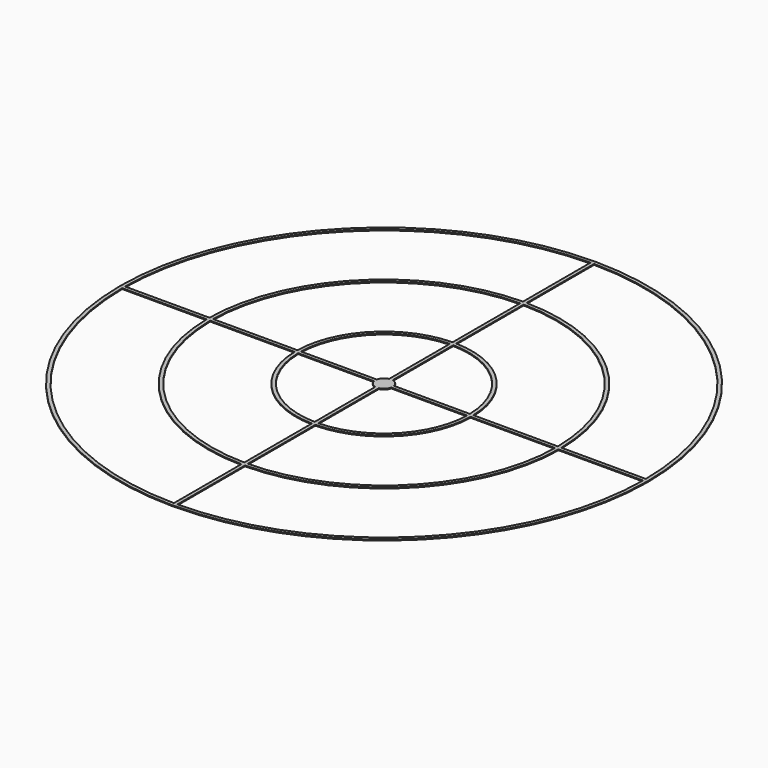
from build123d import *

# Parameters (mm, degrees)
F1_DEPTH = 0.25


with BuildPart() as f1:
    # F0 (on Top) → F1 (new body)
    with BuildSketch(Plane.XY):
        with BuildLine():
            ThreePointArc((-0.5, -73.9983107915), (-52.3259018078, -52.3259018078), (-73.9983107915, -0.5))
            Line((-73.9983107915, -0.5), (-49.9974999375, -0.5))
            Line((-49.9974999375, -0.5), (-48.9974489132, -0.5))
            ThreePointArc((-48.9974489132, -0.5), (-49, 0), (-48.9974489132, 0.5))
            ThreePointArc((-48.9974489132, 0.5), (-34.6482322781, 34.6482322781), (-0.5, 48.9974489132))
            Line((-0.5, 48.9974489132), (-0.5, 49.9974999375))
            ThreePointArc((-0.5, 49.9974999375), (-35.3553390593, 35.3553390593), (-49.9974999375, 0.5))
            Line((-49.9974999375, 0.5), (-73.9983107915, 0.5))
            ThreePointArc((-73.9983107915, 0.5), (-52.3259018078, 52.3259018078), (-0.5, 73.9983107915))
            Line((-0.5, 73.9983107915), (-0.5, 74.9983333148))
            ThreePointArc((-0.5, 74.9983333148), (-53.033008589, 53.033008589), (-74.9983333148, 0.5))
            Line((-74.9983333148, 0.5), (-74.9983333148, -0.5))
            ThreePointArc((-74.9983333148, -0.5), (-53.033008589, -53.033008589), (-0.5, -74.9983333148))
            Line((-0.5, -74.9983333148), (-0.5, -73.9983107915))
        make_face()
        with BuildLine():
            Line((-0.5, -49.9974999375), (-0.5, -73.9983107915))
            ThreePointArc((-0.5, -73.9983107915), (0, -74), (0.5, -73.9983107915))
            Line((0.5, -73.9983107915), (0.5, -49.9974999375))
            ThreePointArc((0.5, -49.9974999375), (0, -50), (-0.5, -49.9974999375))
        make_face()
        with BuildLine():
            ThreePointArc((0.5, -73.9983107915), (0, -74), (-0.5, -73.9983107915))
            Line((-0.5, -73.9983107915), (-0.5, -74.9983333148))
            Line((-0.5, -74.9983333148), (0.5, -74.9983333148))
            Line((0.5, -74.9983333148), (0.5, -73.9983107915))
        make_face()
        with BuildLine():
            Line((-48.9974489132, -0.5), (-49.9974999375, -0.5))
            ThreePointArc((-49.9974999375, -0.5), (-35.3553390593, -35.3553390593), (-0.5, -49.9974999375))
            ThreePointArc((-0.5, -49.9974999375), (0, -50), (0.5, -49.9974999375))
            Line((0.5, -49.9974999375), (0.5, -48.9974489132))
            ThreePointArc((0.5, -48.9974489132), (0, -49), (-0.5, -48.9974489132))
            ThreePointArc((-0.5, -48.9974489132), (-34.6482322781, -34.6482322781), (-48.9974489132, -0.5))
        make_face()
        with BuildLine():
            ThreePointArc((73.9983107915, -0.5), (52.3259018078, -52.3259018078), (0.5, -73.9983107915))
            Line((0.5, -73.9983107915), (0.5, -74.9983333148))
            ThreePointArc((0.5, -74.9983333148), (53.033008589, -53.033008589), (74.9983333148, -0.5))
            Line((74.9983333148, -0.5), (73.9983107915, -0.5))
        make_face()
        with BuildLine():
            ThreePointArc((-48.9974489132, 0.5), (-49, 0), (-48.9974489132, -0.5))
            Line((-48.9974489132, -0.5), (-24.9949994999, -0.5))
            Line((-24.9949994999, -0.5), (-23.9947911014, -0.5))
            ThreePointArc((-23.9947911014, -0.5), (-24, 0), (-23.9947911014, 0.5))
            ThreePointArc((-23.9947911014, 0.5), (-16.9705627485, 16.9705627485), (-0.5, 23.9947911014))
            Line((-0.5, 23.9947911014), (-0.5, 24.9949994999))
            ThreePointArc((-0.5, 24.9949994999), (-17.6776695297, 17.6776695297), (-24.9949994999, 0.5))
            Line((-24.9949994999, 0.5), (-48.9974489132, 0.5))
        make_face()
        with BuildLine():
            Line((49.9974999375, -0.5), (73.9983107915, -0.5))
            ThreePointArc((73.9983107915, -0.5), (74, 0), (73.9983107915, 0.5))
            Line((73.9983107915, 0.5), (49.9974999375, 0.5))
            ThreePointArc((49.9974999375, 0.5), (50, 0), (49.9974999375, -0.5))
        make_face()
        with BuildLine():
            ThreePointArc((73.9983107915, 0.5), (74, 0), (73.9983107915, -0.5))
            Line((73.9983107915, -0.5), (74.9983333148, -0.5))
            Line((74.9983333148, -0.5), (74.9983333148, 0.5))
            Line((74.9983333148, 0.5), (73.9983107915, 0.5))
        make_face()
        with BuildLine():
            Line((0.5, -48.9974489132), (0.5, -49.9974999375))
            ThreePointArc((0.5, -49.9974999375), (35.3553390593, -35.3553390593), (49.9974999375, -0.5))
            Line((49.9974999375, -0.5), (48.9974489132, -0.5))
            ThreePointArc((48.9974489132, -0.5), (34.6482322781, -34.6482322781), (0.5, -48.9974489132))
        make_face()
        with BuildLine():
            ThreePointArc((-74.9983333148, 0.5), (-75, 0), (-74.9983333148, -0.5))
            Line((-74.9983333148, -0.5), (-74.9983333148, 0.5))
        make_face()
        with BuildLine():
            Line((-23.9947911014, -0.5), (-24.9949994999, -0.5))
            ThreePointArc((-24.9949994999, -0.5), (-17.6776695297, -17.6776695297), (-0.5, -24.9949994999))
            Line((-0.5, -24.9949994999), (-0.5, -48.9974489132))
            ThreePointArc((-0.5, -48.9974489132), (0, -49), (0.5, -48.9974489132))
            Line((0.5, -48.9974489132), (0.5, -24.9949994999))
            Line((0.5, -24.9949994999), (0.5, -23.9947911014))
            Line((0.5, -23.9947911014), (0.5, -2.4494897428))
            Line((0.5, -2.4494897428), (0.5, -0.5))
            Line((0.5, -0.5), (2.4494897428, -0.5))
            Line((2.4494897428, -0.5), (23.9947911014, -0.5))
            Line((23.9947911014, -0.5), (24.9949994999, -0.5))
            ThreePointArc((24.9949994999, -0.5), (25, 0), (24.9949994999, 0.5))
            Line((24.9949994999, 0.5), (23.9947911014, 0.5))
            Line((23.9947911014, 0.5), (2.4494897428, 0.5))
            Line((2.4494897428, 0.5), (0.5, 0.5))
            Line((0.5, 0.5), (-0.5, 0.5))
            Line((-0.5, 0.5), (-0.5, -0.5))
            Line((-0.5, -0.5), (-0.5, -2.4494897428))
            Line((-0.5, -2.4494897428), (-0.5, -23.9947911014))
            ThreePointArc((-0.5, -23.9947911014), (-16.9705627485, -16.9705627485), (-23.9947911014, -0.5))
        make_face()
        with BuildLine():
            ThreePointArc((0.5, 73.9983107915), (52.3259018078, 52.3259018078), (73.9983107915, 0.5))
            Line((73.9983107915, 0.5), (74.9983333148, 0.5))
            ThreePointArc((74.9983333148, 0.5), (53.033008589, 53.033008589), (0.5, 74.9983333148))
            Line((0.5, 74.9983333148), (0.5, 73.9983107915))
        make_face()
        with BuildLine():
            Line((48.9974489132, -0.5), (49.9974999375, -0.5))
            ThreePointArc((49.9974999375, -0.5), (50, 0), (49.9974999375, 0.5))
            Line((49.9974999375, 0.5), (48.9974489132, 0.5))
            ThreePointArc((48.9974489132, 0.5), (49, 0), (48.9974489132, -0.5))
        make_face()
        with BuildLine():
            Line((-0.5, 49.9974999375), (-0.5, 48.9974489132))
            ThreePointArc((-0.5, 48.9974489132), (0, 49), (0.5, 48.9974489132))
            Line((0.5, 48.9974489132), (0.5, 49.9974999375))
            ThreePointArc((0.5, 49.9974999375), (0, 50), (-0.5, 49.9974999375))
        make_face()
        with BuildLine():
            ThreePointArc((0.5, 48.9974489132), (0, 49), (-0.5, 48.9974489132))
            Line((-0.5, 48.9974489132), (-0.5, 24.9949994999))
            Line((-0.5, 24.9949994999), (-0.5, 23.9947911014))
            ThreePointArc((-0.5, 23.9947911014), (0, 24), (0.5, 23.9947911014))
            ThreePointArc((0.5, 23.9947911014), (16.9705627485, 16.9705627485), (23.9947911014, 0.5))
            Line((23.9947911014, 0.5), (24.9949994999, 0.5))
            ThreePointArc((24.9949994999, 0.5), (17.6776695297, 17.6776695297), (0.5, 24.9949994999))
            Line((0.5, 24.9949994999), (0.5, 48.9974489132))
        make_face()
        with BuildLine():
            ThreePointArc((-23.9947911014, 0.5), (-24, 0), (-23.9947911014, -0.5))
            Line((-23.9947911014, -0.5), (-2.4494897428, -0.5))
            Line((-2.4494897428, -0.5), (-0.5, -0.5))
            Line((-0.5, -0.5), (-0.5, 0.5))
            Line((-0.5, 0.5), (-2.4494897428, 0.5))
            Line((-2.4494897428, 0.5), (-23.9947911014, 0.5))
        make_face()
        with BuildLine():
            Line((0.5, 49.9974999375), (0.5, 73.9983107915))
            ThreePointArc((0.5, 73.9983107915), (0, 74), (-0.5, 73.9983107915))
            Line((-0.5, 73.9983107915), (-0.5, 49.9974999375))
            ThreePointArc((-0.5, 49.9974999375), (0, 50), (0.5, 49.9974999375))
        make_face()
        with BuildLine():
            ThreePointArc((-0.5, 73.9983107915), (0, 74), (0.5, 73.9983107915))
            Line((0.5, 73.9983107915), (0.5, 74.9983333148))
            Line((0.5, 74.9983333148), (-0.5, 74.9983333148))
            Line((-0.5, 74.9983333148), (-0.5, 73.9983107915))
        make_face()
        with BuildLine():
            Line((48.9974489132, 0.5), (49.9974999375, 0.5))
            ThreePointArc((49.9974999375, 0.5), (35.3553390593, 35.3553390593), (0.5, 49.9974999375))
            Line((0.5, 49.9974999375), (0.5, 48.9974489132))
            ThreePointArc((0.5, 48.9974489132), (34.6482322781, 34.6482322781), (48.9974489132, 0.5))
        make_face()
        with BuildLine():
            Line((24.9949994999, -0.5), (48.9974489132, -0.5))
            ThreePointArc((48.9974489132, -0.5), (49, 0), (48.9974489132, 0.5))
            Line((48.9974489132, 0.5), (24.9949994999, 0.5))
            ThreePointArc((24.9949994999, 0.5), (25, 0), (24.9949994999, -0.5))
        make_face()
        with BuildLine():
            Line((0.5, -23.9947911014), (0.5, -24.9949994999))
            ThreePointArc((0.5, -24.9949994999), (17.6776695297, -17.6776695297), (24.9949994999, -0.5))
            Line((24.9949994999, -0.5), (23.9947911014, -0.5))
            ThreePointArc((23.9947911014, -0.5), (16.9705627485, -16.9705627485), (0.5, -23.9947911014))
        make_face()
        with BuildLine():
            ThreePointArc((0.5, 74.9983333148), (0, 75), (-0.5, 74.9983333148))
            Line((-0.5, 74.9983333148), (0.5, 74.9983333148))
        make_face()
        with BuildLine():
            Line((-0.5, -0.5), (-2.4494897428, -0.5))
            ThreePointArc((-2.4494897428, -0.5), (-1.767766953, -1.767766953), (-0.5, -2.4494897428))
            Line((-0.5, -2.4494897428), (-0.5, -0.5))
        make_face()
        with BuildLine():
            ThreePointArc((0.5, 23.9947911014), (0, 24), (-0.5, 23.9947911014))
            Line((-0.5, 23.9947911014), (-0.5, 2.4494897428))
            Line((-0.5, 2.4494897428), (-0.5, 0.5))
            Line((-0.5, 0.5), (0.5, 0.5))
            Line((0.5, 0.5), (0.5, 2.4494897428))
            Line((0.5, 2.4494897428), (0.5, 23.9947911014))
        make_face()
        with BuildLine():
            ThreePointArc((-0.5, 2.4494897428), (-1.767766953, 1.767766953), (-2.4494897428, 0.5))
            Line((-2.4494897428, 0.5), (-0.5, 0.5))
            Line((-0.5, 0.5), (-0.5, 2.4494897428))
        make_face()
        with BuildLine():
            Line((0.5, -0.5), (0.5, -2.4494897428))
            ThreePointArc((0.5, -2.4494897428), (1.767766953, -1.767766953), (2.4494897428, -0.5))
            Line((2.4494897428, -0.5), (0.5, -0.5))
        make_face()
        with BuildLine():
            ThreePointArc((2.4494897428, 0.5), (1.767766953, 1.767766953), (0.5, 2.4494897428))
            Line((0.5, 2.4494897428), (0.5, 0.5))
            Line((0.5, 0.5), (2.4494897428, 0.5))
        make_face()
    extrude(amount=F1_DEPTH)


solid = f1.part
